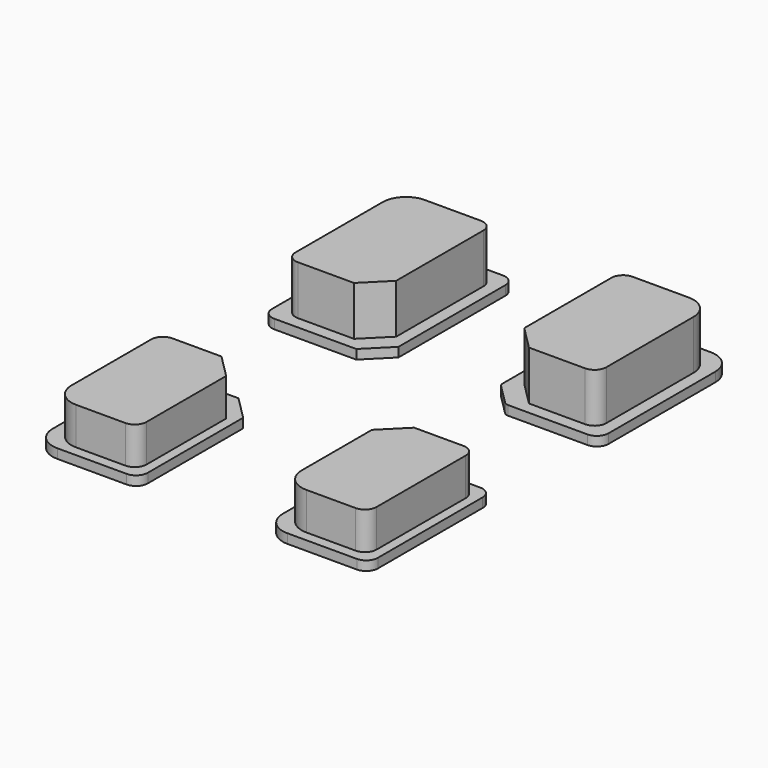
from build123d import *

# Parameters (mm, degrees)
F0_W       = 7.8
F0_H       = 12.3
F1_DEPTH   = 5
F0_W_2     = 10
F0_H_2     = 14.4
F2_DEPTH   = 0.8
F3_R       = 1
F3_2_R     = 1
F4_R       = 2
F4_2_R     = 2
F5_DEPTH   = 0.8
F6_SIZE    = 2
F6_2_SIZE  = 2
F7_R       = 0.5
F8_R       = 2
F9_R       = 1
F10_W      = 7.2
F10_H      = 11.5
F11_DEPTH  = 4
F10_W_2    = 8.9209638536
F10_H_2    = 13.1787001155
F12_DEPTH  = 0.8
F13_R      = 2
F13_2_R    = 2
F14_R      = 1
F14_2_R    = 1
F15_DEPTH  = 3.2
F16_DEPTH  = 2.4
F17_DEPTH  = 3
F18_DEPTH  = 3
F19_SIZE   = 2
F19_2_SIZE = 2


with BuildPart() as f1:
    # F0 (on Top) → F1 (new body)
    with BuildSketch(Plane.XY):
        with Locations((-34.8363173068, 6.15)):
            Rectangle(F0_W, F0_H)
        Polygon((-38.0835977137, 0.6249411381), (-38.0835977137, 11.7249411381), (-31.5835977137, 11.7249411381), (-31.5835977137, 2.2546383552), (-31.5835977137, 0.6249411381), (-33.3403423429, 0.6249411381), align=None, mode=Mode.SUBTRACT)
        Polygon((-31.5835977137, 11.7249411381), (-38.0835977137, 11.7249411381), (-38.0835977137, 0.6249411381), (-33.3403423429, 0.6249411381), (-31.5835977137, 2.2546383552), align=None)
        Polygon((-31.5835977137, 0.6249411381), (-31.5835977137, 2.2546383552), (-33.3403423429, 0.6249411381), align=None)
    extrude(amount=F1_DEPTH)

    # F0 (on Top) → F2 (join)
    with BuildSketch(Plane.XY):
        with Locations((-34.9024849355, 6.1506106358)):
            Rectangle(F0_W_2, F0_H_2)
        with Locations((-34.8363173068, 6.15)):
            Rectangle(F0_W, F0_H, mode=Mode.SUBTRACT)
    extrude(amount=F2_DEPTH)

    # F3
    f3_edges = [f1.edges().sort_by_distance(p)[0] for p in [
        (-38.736317, 0, 2.9),
        (-39.902485, -1.049389, 0.4),
        (-29.902485, 13.350611, 0.4),
        (-30.936317, 12.3, 2.9),
    ]]
    fillet(f3_edges, radius=F3_R)

    # F4
    f4_edges = [f1.edges().sort_by_distance(p)[0] for p in [
        (-39.902485, 13.350611, 0.4),
        (-38.736317, 12.3, 2.9),
    ]]
    fillet(f4_edges, radius=F4_R)

    # F6
    f6_edges = [f1.edges().sort_by_distance(p)[0] for p in [
        (-29.902485, -1.049389, 0.4),
        (-30.936317, 0, 2.9),
    ]]
    chamfer(f6_edges, length=F6_SIZE)

    # F0 (on Top) → F16 (cut)
    with BuildSketch(Plane.XY):
        Polygon((-31.5835977137, 11.7249411381), (-38.0835977137, 11.7249411381), (-38.0835977137, 0.6249411381), (-33.3403423429, 0.6249411381), (-31.5835977137, 2.2546383552), align=None)
    extrude(amount=F16_DEPTH, mode=Mode.SUBTRACT)


with BuildPart() as f1b:
    # F0 (on Top) → F1, piece 2 (new body)
    with BuildSketch(Plane.XY):
        with Locations((-16.1042231411, 6.15)):
            Rectangle(F0_W, F0_H)
        Polygon((-19.3634564057, 2.4356972507), (-19.3634564057, 11.6938437534), (-12.8634564057, 11.6938437534), (-12.8634564057, 0.5938437534), (-17.6548053763, 0.5938437534), (-19.3634564057, 0.5938437534), align=None, mode=Mode.SUBTRACT)
        Polygon((-12.8634564057, 11.6938437534), (-19.3634564057, 11.6938437534), (-19.3634564057, 2.4356972507), (-17.6548053763, 0.5938437534), (-12.8634564057, 0.5938437534), align=None)
        Polygon((-17.6548053763, 0.5938437534), (-19.3634564057, 2.4356972507), (-19.3634564057, 0.5938437534), align=None)
    extrude(amount=F1_DEPTH)

    # F3#2
    f3_2_edges = [f1b.edges().sort_by_distance(p)[0] for p in [
        (-12.204223, 0, 2.5),
        (-20.004223, 12.3, 2.5),
    ]]
    fillet(f3_2_edges, radius=F3_2_R)

    # F4#2
    f4_2_edges = [f1b.edges().sort_by_distance(p)[0] for p in [
        (-12.204223, 12.3, 2.5),
    ]]
    fillet(f4_2_edges, radius=F4_2_R)

    # F0 (on Top) → F5 (join)
    with BuildSketch(Plane.XY):
        with Locations((-16.1703907698, 6.1506106358)):
            Rectangle(F0_W_2, F0_H_2)
        with Locations((-16.1042231411, 6.15)):
            Rectangle(F0_W, F0_H, mode=Mode.SUBTRACT)
        with Locations((-16.1042231411, 6.15)):
            Rectangle(F0_W, F0_H)
        Polygon((-19.3634564057, 2.4356972507), (-19.3634564057, 11.6938437534), (-12.8634564057, 11.6938437534), (-12.8634564057, 0.5938437534), (-17.6548053763, 0.5938437534), (-19.3634564057, 0.5938437534), align=None, mode=Mode.SUBTRACT)
        Polygon((-12.8634564057, 11.6938437534), (-19.3634564057, 11.6938437534), (-19.3634564057, 2.4356972507), (-17.6548053763, 0.5938437534), (-12.8634564057, 0.5938437534), align=None)
    extrude(amount=F5_DEPTH)

    # F6#2
    f6_2_edges = [f1b.edges().sort_by_distance(p)[0] for p in [
        (-21.170391, -1.049389, 0.4),
        (-20.004223, 0, 2.9),
    ]]
    chamfer(f6_2_edges, length=F6_2_SIZE)

    # F7
    f7_edges = [f1b.edges().sort_by_distance(p)[0] for p in [
        (-21.170391, 0.950611, 0.4),
        (-19.170391, -1.049389, 0.4),
    ]]
    fillet(f7_edges, radius=F7_R)

    # F8
    f8_edges = [f1b.edges().sort_by_distance(p)[0] for p in [
        (-11.170391, 13.350611, 0.4),
    ]]
    fillet(f8_edges, radius=F8_R)

    # F9
    f9_edges = [f1b.edges().sort_by_distance(p)[0] for p in [
        (-11.170391, -1.049389, 0.4),
        (-21.170391, 13.350611, 0.4),
    ]]
    fillet(f9_edges, radius=F9_R)

    # F0 (on Top) → F15 (cut)
    with BuildSketch(Plane.XY):
        Polygon((-12.8634564057, 11.6938437534), (-19.3634564057, 11.6938437534), (-19.3634564057, 2.4356972507), (-17.6548053763, 0.5938437534), (-12.8634564057, 0.5938437534), align=None)
    extrude(amount=F15_DEPTH, mode=Mode.SUBTRACT)


with BuildPart() as f11:
    # F10 (on Top) → F11 (new body)
    with BuildSketch(Plane.XY):
        with Locations((-36.0041396379, -18.056700483)):
            Rectangle(F10_W, F10_H)
        Polygon((-38.9729559064, -23.2622586191), (-38.9729559064, -12.8622586191), (-34.2715643346, -12.8622586191), (-33.0729559064, -12.8622586191), (-33.0729559064, -14.0329562128), (-33.0729559064, -23.2622586191), align=None, mode=Mode.SUBTRACT)
        Polygon((-34.2715643346, -12.8622586191), (-38.9729559064, -12.8622586191), (-38.9729559064, -23.2622586191), (-33.0729559064, -23.2622586191), (-33.0729559064, -14.0329562128), align=None)
        Polygon((-33.0729559064, -12.8622586191), (-34.2715643346, -12.8622586191), (-33.0729559064, -14.0329562128), align=None)
    extrude(amount=F11_DEPTH)

    # F10 (on Top) → F12 (join)
    with BuildSketch(Plane.XY):
        with Locations((-36.0536258668, -18.0959303398)):
            Rectangle(F10_W_2, F10_H_2)
        with Locations((-36.0041396379, -18.056700483)):
            Rectangle(F10_W, F10_H, mode=Mode.SUBTRACT)
        with Locations((-36.0041396379, -18.056700483)):
            Rectangle(F10_W, F10_H)
        Polygon((-38.9729559064, -23.2622586191), (-38.9729559064, -12.8622586191), (-34.2715643346, -12.8622586191), (-33.0729559064, -12.8622586191), (-33.0729559064, -14.0329562128), (-33.0729559064, -23.2622586191), align=None, mode=Mode.SUBTRACT)
    extrude(amount=F12_DEPTH)

    # F13
    f13_edges = [f11.edges().sort_by_distance(p)[0] for p in [
        (-39.60414, -23.8067, 2.4),
        (-40.514108, -24.68528, 0.4),
    ]]
    fillet(f13_edges, radius=F13_R)

    # F14
    f14_edges = [f11.edges().sort_by_distance(p)[0] for p in [
        (-32.40414, -23.8067, 2.4),
        (-31.593144, -24.68528, 0.4),
        (-39.60414, -12.3067, 2.4),
        (-40.514108, -11.50658, 0.4),
    ]]
    fillet(f14_edges, radius=F14_R)

    # F10 (on Top) → F17 (cut)
    with BuildSketch(Plane.XY):
        Polygon((-34.2715643346, -12.8622586191), (-38.9729559064, -12.8622586191), (-38.9729559064, -23.2622586191), (-33.0729559064, -23.2622586191), (-33.0729559064, -14.0329562128), align=None)
    extrude(amount=F17_DEPTH, mode=Mode.SUBTRACT)

    # F19
    f19_edges = [f11.edges().sort_by_distance(p)[0] for p in [
        (-32.40414, -12.3067, 2.4),
        (-31.593144, -11.50658, 0.4),
    ]]
    chamfer(f19_edges, length=F19_SIZE)


with BuildPart() as f11b:
    # F10 (on Top) → F11, piece 2 (new body)
    with BuildSketch(Plane.XY):
        with Locations((-16.3590158954, -18.056700483)):
            Rectangle(F10_W, F10_H)
        Polygon((-19.2590169609, -14.0329562128), (-19.2590169609, -12.8423916459), (-18.0903207511, -12.8423916459), (-13.3590169609, -12.8423916459), (-13.3590169609, -23.2423916459), (-19.2590169609, -23.2423916459), align=None, mode=Mode.SUBTRACT)
        Polygon((-18.0903207511, -12.8423916459), (-19.2590169609, -12.8423916459), (-19.2590169609, -14.0329562128), align=None)
        Polygon((-13.3590169609, -12.8423916459), (-18.0903207511, -12.8423916459), (-19.2590169609, -14.0329562128), (-19.2590169609, -23.2423916459), (-13.3590169609, -23.2423916459), align=None)
    extrude(amount=F11_DEPTH)

    # F10 (on Top) → F12, piece 2 (join)
    with BuildSketch(Plane.XY):
        with Locations((-16.4085021242, -18.0959303398)):
            Rectangle(F10_W_2, F10_H_2)
        with Locations((-16.3590158954, -18.056700483)):
            Rectangle(F10_W, F10_H, mode=Mode.SUBTRACT)
        with Locations((-16.3590158954, -18.056700483)):
            Rectangle(F10_W, F10_H)
        Polygon((-19.2590169609, -14.0329562128), (-19.2590169609, -12.8423916459), (-18.0903207511, -12.8423916459), (-13.3590169609, -12.8423916459), (-13.3590169609, -23.2423916459), (-19.2590169609, -23.2423916459), align=None, mode=Mode.SUBTRACT)
    extrude(amount=F12_DEPTH)

    # F13#2
    f13_2_edges = [f11b.edges().sort_by_distance(p)[0] for p in [
        (-19.959016, -23.8067, 2.4),
        (-20.868984, -24.68528, 0.4),
    ]]
    fillet(f13_2_edges, radius=F13_2_R)

    # F14#2
    f14_2_edges = [f11b.edges().sort_by_distance(p)[0] for p in [
        (-12.759016, -23.8067, 2.4),
        (-11.94802, -24.68528, 0.4),
        (-12.759016, -12.3067, 2.4),
        (-11.94802, -11.50658, 0.4),
    ]]
    fillet(f14_2_edges, radius=F14_2_R)

    # F10 (on Top) → F18 (cut)
    with BuildSketch(Plane.XY):
        Polygon((-13.3590169609, -12.8423916459), (-18.0903207511, -12.8423916459), (-19.2590169609, -14.0329562128), (-19.2590169609, -23.2423916459), (-13.3590169609, -23.2423916459), align=None)
    extrude(amount=F18_DEPTH, mode=Mode.SUBTRACT)

    # F19#2
    f19_2_edges = [f11b.edges().sort_by_distance(p)[0] for p in [
        (-19.959016, -12.3067, 2.4),
        (-20.868984, -11.50658, 0.4),
    ]]
    chamfer(f19_2_edges, length=F19_2_SIZE)


solid = Compound([f1.part, f1b.part, f11.part, f11b.part])
